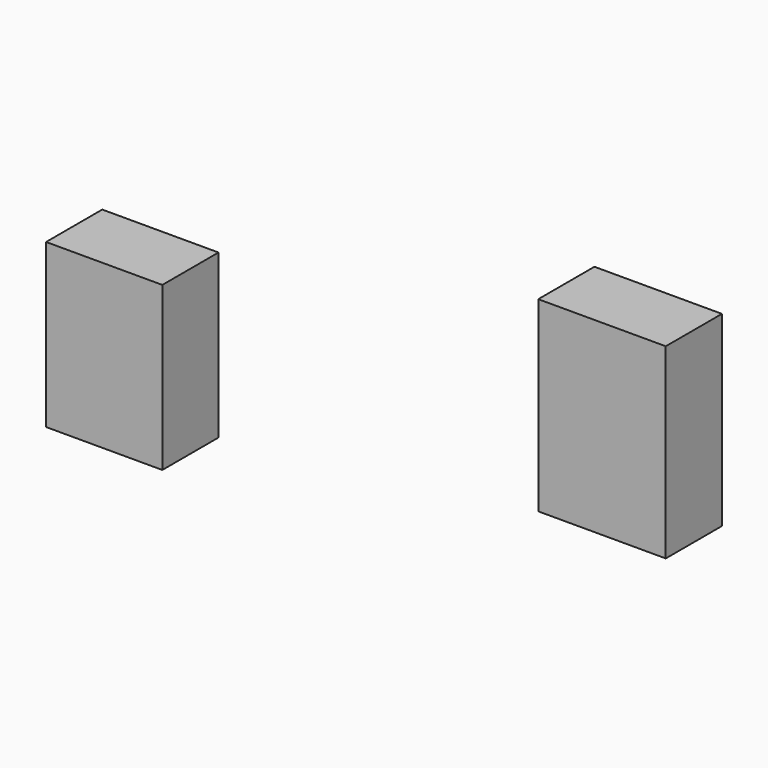
from build123d import *

# Parameters (mm, degrees)
F0_W     = 41.3896143436
F0_H     = 58.0107783899
F1_DEPTH = 25
F0_W_2   = 45.3950315714
F0_H_2   = 66.5103532374


# Not quite as in the source:
# - the program builds the solid bodies; features that only make, move or delete a surface that nothing else refers to are left out


with BuildPart() as f1:
    # F0 (on Front) → F1 (new body)
    with BuildSketch(Plane.XZ):
        with Locations((-125.1701712608, 24.4488511235)):
            Rectangle(F0_W, F0_H)
    extrude(amount=F1_DEPTH)


with BuildPart() as f1b:
    # F0 (on Front) → F1, piece 2 (new body)
    with BuildSketch(Plane.XZ):
        with Locations((52.0707890391, 59.2583417892)):
            Rectangle(F0_W_2, F0_H_2)
    extrude(amount=F1_DEPTH)


solid = Compound([f1.part, f1b.part])
